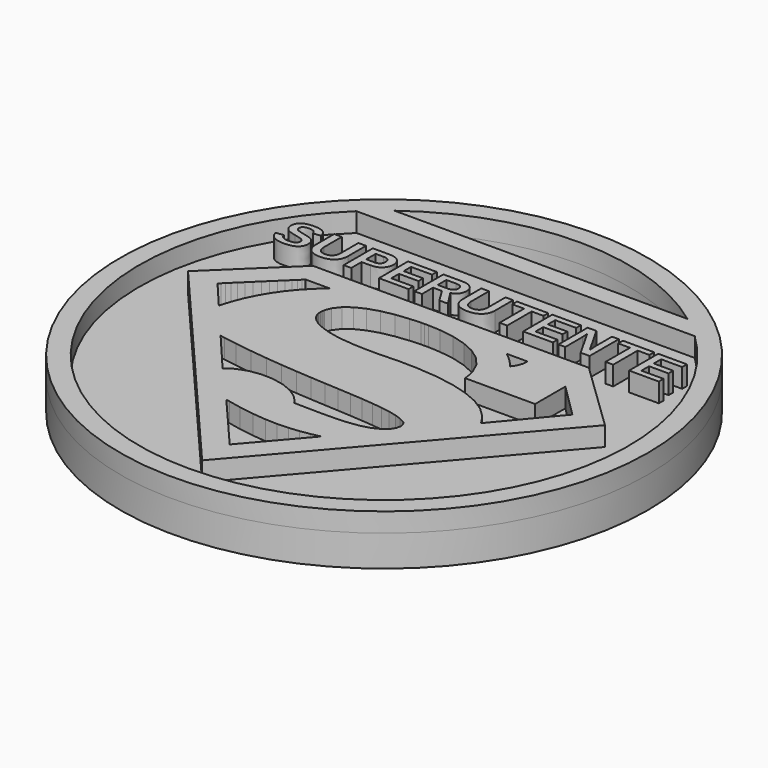
from build123d import *

# Parameters (mm, degrees)
F0_R         = 11
F0_TEXT_SIZE = 2.2071271815
F1_DEPTH     = 1.3
F2_DEPTH     = 0.8


# Not quite as in the source:
# - a feature names something its author has since deleted; it is built from what else it names
# - Text() gives the source's letters only with a copy of the font that has no kerning and outlines rounded to 1/6400 em; it was checked with that copy


with BuildPart() as f1:
    # F0 (on Top) → F1 (new body)
    with BuildSketch(Plane.XY):
        with Locations((0, 3)):
            Circle(F0_R)
        with BuildLine():
            ThreePointArc((7.048873348, 10.3724747896), (0, -7.2), (-7.048873348, 10.3724747896))
            Line((-7.048873348, 10.3724747896), (7.048873348, 10.3724747896))
        make_face(mode=Mode.SUBTRACT)
        with BuildLine():
            Line((6.1033309693, 11.1724752113), (-6.1033309693, 11.1724752113))
            ThreePointArc((-6.1033309693, 11.1724752113), (0, 13.2), (6.1033309693, 11.1724752113))
        make_face(mode=Mode.SUBTRACT)
        with BuildLine():
            Line((7.048873348, 10.3724747896), (-7.048873348, 10.3724747896))
            ThreePointArc((-7.048873348, 10.3724747896), (0, -7.2), (7.048873348, 10.3724747896))
        make_face()
        Polygon((8.687503, 3.64583), (3e-06, -6.47917), (-8.687503, 3.64583), (-5.749997, 6.47917), (5.750003, 6.47917), align=None, mode=Mode.SUBTRACT)
        with BuildLine():
            add(Edge.make_bspline(
                [(-6.856384511, 7.7478548692), (-6.8272435349, 7.6750886449), (-6.8272435349, 7.5802511488)],
                knots=[0, 0, 0, 1, 1, 1], degree=2))
            add(Edge.make_bspline(
                [(-6.8272435349, 7.5802511488), (-6.8272435349, 7.3571243853), (-6.9927780735, 7.2390085947)],
                knots=[0, 0, 0, 1, 1, 1], degree=2))
            add(Edge.make_bspline(
                [(-6.9927780735, 7.2390085947), (-7.1583126121, 7.1208928042), (-7.4783460534, 7.1208928042)],
                knots=[0, 0, 0, 1, 1, 1], degree=2))
            add(Edge.make_bspline(
                [(-7.4783460534, 7.1208928042), (-7.7704455414, 7.1208928042), (-7.9363249436, 7.2245243226)],
                knots=[0, 0, 0, 1, 1, 1], degree=2))
            add(Edge.make_bspline(
                [(-7.9363249436, 7.2245243226), (-8.1022043458, 7.3281558411), (-8.1497955257, 7.5381777869)],
                knots=[0, 0, 0, 1, 1, 1], degree=2))
            Line((-8.1497955257, 7.5381777869), (-7.8425220384, 7.5888727394))
            add(Edge.make_bspline(
                [(-7.8425220384, 7.5888727394), (-7.8111394488, 7.4681704716), (-7.720612748, 7.4136820193)],
                knots=[0, 0, 0, 1, 1, 1], degree=2))
            add(Edge.make_bspline(
                [(-7.720612748, 7.4136820193), (-7.6300860472, 7.3591935671), (-7.4697244629, 7.3591935671)],
                knots=[0, 0, 0, 1, 1, 1], degree=2))
            add(Edge.make_bspline(
                [(-7.4697244629, 7.3591935671), (-7.1365862039, 7.3591935671), (-7.1365862039, 7.5619733769)],
                knots=[0, 0, 0, 1, 1, 1], degree=2))
            add(Edge.make_bspline(
                [(-7.1365862039, 7.5619733769), (-7.1365862039, 7.6264628742), (-7.174866066, 7.6685362361)],
                knots=[0, 0, 0, 1, 1, 1], degree=2))
            add(Edge.make_bspline(
                [(-7.174866066, 7.6685362361), (-7.213145928, 7.710609598), (-7.2826359479, 7.7385435514)],
                knots=[0, 0, 0, 1, 1, 1], degree=2))
            add(Edge.make_bspline(
                [(-7.2826359479, 7.7385435514), (-7.3521259677, 7.7664775048), (-7.5493879596, 7.8064816849)],
                knots=[0, 0, 0, 1, 1, 1], degree=2))
            add(Edge.make_bspline(
                [(-7.5493879596, 7.8064816849), (-7.7197505889, 7.8464858651), (-7.7864816998, 7.8706263186)],
                knots=[0, 0, 0, 1, 1, 1], degree=2))
            add(Edge.make_bspline(
                [(-7.7864816998, 7.8706263186), (-7.8532128107, 7.8947667722), (-7.9071839675, 7.9277012481)],
                knots=[0, 0, 0, 1, 1, 1], degree=2))
            add(Edge.make_bspline(
                [(-7.9071839675, 7.9277012481), (-7.9611551244, 7.960635724), (-7.9987452592, 8.0070198812)],
                knots=[0, 0, 0, 1, 1, 1], degree=2))
            add(Edge.make_bspline(
                [(-7.9987452592, 8.0070198812), (-8.036335394, 8.0534040384), (-8.057372075, 8.115824354)],
                knots=[0, 0, 0, 1, 1, 1], degree=2))
            add(Edge.make_bspline(
                [(-8.057372075, 8.115824354), (-8.0784087559, 8.1782446696), (-8.0784087559, 8.2592876208)],
                knots=[0, 0, 0, 1, 1, 1], degree=2))
            add(Edge.make_bspline(
                [(-8.0784087559, 8.2592876208), (-8.0784087559, 8.4648263395), (-7.9237374214, 8.5743205396)],
                knots=[0, 0, 0, 1, 1, 1], degree=2))
            add(Edge.make_bspline(
                [(-7.9237374214, 8.5743205396), (-7.7690660869, 8.6838147396), (-7.4738628264, 8.6838147396)],
                knots=[0, 0, 0, 1, 1, 1], degree=2))
            add(Edge.make_bspline(
                [(-7.4738628264, 8.6838147396), (-7.1914195198, 8.6838147396), (-7.049853003, 8.5953572205)],
                knots=[0, 0, 0, 1, 1, 1], degree=2))
            add(Edge.make_bspline(
                [(-7.049853003, 8.5953572205), (-6.9082864861, 8.5068997014), (-6.8672477151, 8.3034301644)],
                knots=[0, 0, 0, 1, 1, 1], degree=2))
            Line((-6.8672477151, 8.3034301644), (-7.1755557932, 8.2613568025))
            add(Edge.make_bspline(
                [(-7.1755557932, 8.2613568025), (-7.1990065195, 8.3592980712), (-7.2717727438, 8.4089584328)],
                knots=[0, 0, 0, 1, 1, 1], degree=2))
            add(Edge.make_bspline(
                [(-7.2717727438, 8.4089584328), (-7.3445389681, 8.4586187943), (-7.4804152352, 8.4586187943)],
                knots=[0, 0, 0, 1, 1, 1], degree=2))
            add(Edge.make_bspline(
                [(-7.4804152352, 8.4586187943), (-7.7690660869, 8.4586187943), (-7.7690660869, 8.2775653927)],
                knots=[0, 0, 0, 1, 1, 1], degree=2))
            add(Edge.make_bspline(
                [(-7.7690660869, 8.2775653927), (-7.7690660869, 8.2182488497), (-7.7383732245, 8.1804862831)],
                knots=[0, 0, 0, 1, 1, 1], degree=2))
            add(Edge.make_bspline(
                [(-7.7383732245, 8.1804862831), (-7.7076803621, 8.1427237165), (-7.6473292283, 8.115824354)],
                knots=[0, 0, 0, 1, 1, 1], degree=2))
            add(Edge.make_bspline(
                [(-7.6473292283, 8.115824354), (-7.5869780944, 8.0889249914), (-7.4028209202, 8.0499554021)],
                knots=[0, 0, 0, 1, 1, 1], degree=2))
            add(Edge.make_bspline(
                [(-7.4028209202, 8.0499554021), (-7.1841773838, 8.0037436768), (-7.0898571831, 7.9644292239)],
                knots=[0, 0, 0, 1, 1, 1], degree=2))
            add(Edge.make_bspline(
                [(-7.0898571831, 7.9644292239), (-6.9955369825, 7.9251147709), (-6.9405312348, 7.8728679322)],
                knots=[0, 0, 0, 1, 1, 1], degree=2))
            add(Edge.make_bspline(
                [(-6.9405312348, 7.8728679322), (-6.885525487, 7.8206210934), (-6.856384511, 7.7478548692)],
                knots=[0, 0, 0, 1, 1, 1], degree=2))
        make_face(mode=Mode.SUBTRACT)
        with BuildLine():
            add(Edge.make_bspline(
                [(-5.4602041368, 7.279874934), (-5.6384986295, 7.1208928042), (-5.961980707, 7.1208928042)],
                knots=[0, 0, 0, 1, 1, 1], degree=2))
            add(Edge.make_bspline(
                [(-5.961980707, 7.1208928042), (-6.2754617395, 7.1208928042), (-6.442030869, 7.2740122524)],
                knots=[0, 0, 0, 1, 1, 1], degree=2))
            add(Edge.make_bspline(
                [(-6.442030869, 7.2740122524), (-6.6085999985, 7.4271317006), (-6.6085999985, 7.7116441889)],
                knots=[0, 0, 0, 1, 1, 1], degree=2))
            Line((-6.6085999985, 7.7116441889), (-6.6085999985, 8.6610537405))
            Line((-6.6085999985, 8.6610537405), (-6.2906357389, 8.6610537405))
            Line((-6.2906357389, 8.6610537405), (-6.2906357389, 7.7364743696))
            add(Edge.make_bspline(
                [(-6.2906357389, 7.7364743696), (-6.2906357389, 7.5564555589), (-6.2049371288, 7.4631699491)],
                knots=[0, 0, 0, 1, 1, 1], degree=2))
            add(Edge.make_bspline(
                [(-6.2049371288, 7.4631699491), (-6.1192385187, 7.3698843393), (-5.9533591165, 7.3698843393)],
                knots=[0, 0, 0, 1, 1, 1], degree=2))
            add(Edge.make_bspline(
                [(-5.9533591165, 7.3698843393), (-5.7829964871, 7.3698843393), (-5.6914351955, 7.4674807444)],
                knots=[0, 0, 0, 1, 1, 1], degree=2))
            add(Edge.make_bspline(
                [(-5.6914351955, 7.4674807444), (-5.5998739038, 7.5650771495), (-5.5998739038, 7.7471651419)],
                knots=[0, 0, 0, 1, 1, 1], degree=2))
            Line((-5.5998739038, 7.7471651419), (-5.5998739038, 8.6610537405))
            Line((-5.5998739038, 8.6610537405), (-5.2819096442, 8.6610537405))
            Line((-5.2819096442, 8.6610537405), (-5.2819096442, 7.7278527791))
            add(Edge.make_bspline(
                [(-5.2819096442, 7.7278527791), (-5.2819096442, 7.4388570638), (-5.4602041368, 7.279874934)],
                knots=[0, 0, 0, 1, 1, 1], degree=2))
        make_face(mode=Mode.SUBTRACT)
        with BuildLine():
            add(Edge.make_bspline(
                [(-3.8974546332, 8.5355233821), (-3.7503702984, 8.4099930236), (-3.7503702984, 8.1803138513)],
                knots=[0, 0, 0, 1, 1, 1], degree=2))
            add(Edge.make_bspline(
                [(-3.7503702984, 8.1803138513), (-3.7503702984, 8.0337468119), (-3.8171014093, 7.9185623621)],
                knots=[0, 0, 0, 1, 1, 1], degree=2))
            add(Edge.make_bspline(
                [(-3.8171014093, 7.9185623621), (-3.8838325202, 7.8033779123), (-4.0083282877, 7.7402678695)],
                knots=[0, 0, 0, 1, 1, 1], degree=2))
            add(Edge.make_bspline(
                [(-4.0083282877, 7.7402678695), (-4.1328240553, 7.6771578266), (-4.3042212755, 7.6771578266)],
                knots=[0, 0, 0, 1, 1, 1], degree=2))
            Line((-4.3042212755, 7.6771578266), (-4.6815020781, 7.6771578266))
            Line((-4.6815020781, 7.6771578266), (-4.6815020781, 7.1426192124))
            Line((-4.6815020781, 7.1426192124), (-4.9994663377, 7.1426192124))
            Line((-4.9994663377, 7.1426192124), (-4.9994663377, 8.6610537405))
            Line((-4.9994663377, 8.6610537405), (-4.3173260932, 8.6610537405))
            add(Edge.make_bspline(
                [(-4.3173260932, 8.6610537405), (-4.0445389681, 8.6610537405), (-3.8974546332, 8.5355233821)],
                knots=[0, 0, 0, 1, 1, 1], degree=2))
        make_face(mode=Mode.SUBTRACT)
        Polygon((-2.2888382679, 7.1426192124), (-3.5272435349, 7.1426192124), (-3.5272435349, 8.6610537405), (-2.3329808115, 8.6610537405), (-2.3329808115, 8.4155108416), (-3.2092792753, 8.4155108416), (-3.2092792753, 8.0337468119), (-2.3988497633, 8.0337468119), (-2.3988497633, 7.788203913), (-3.2092792753, 7.788203913), (-3.2092792753, 7.3885069749), (-2.2888382679, 7.3885069749), align=None, mode=Mode.SUBTRACT)
        with BuildLine():
            Line((-0.6538398354, 7.1426192124), (-1.0118082752, 7.1426192124))
            Line((-1.0118082752, 7.1426192124), (-1.364258897, 7.7192311885))
            Line((-1.364258897, 7.7192311885), (-1.7370564725, 7.7192311885))
            Line((-1.7370564725, 7.7192311885), (-1.7370564725, 7.1426192124))
            Line((-1.7370564725, 7.1426192124), (-2.0550207321, 7.1426192124))
            Line((-2.0550207321, 7.1426192124), (-2.0550207321, 8.6610537405))
            Line((-2.0550207321, 8.6610537405), (-1.2963207634, 8.6610537405))
            add(Edge.make_bspline(
                [(-1.2963207634, 8.6610537405), (-1.0245682292, 8.6610537405), (-0.876966599, 8.5441449726)],
                knots=[0, 0, 0, 1, 1, 1], degree=2))
            add(Edge.make_bspline(
                [(-0.876966599, 8.5441449726), (-0.7293649687, 8.4272362047), (-0.7293649687, 8.2085926683)],
                knots=[0, 0, 0, 1, 1, 1], degree=2))
            add(Edge.make_bspline(
                [(-0.7293649687, 8.2085926683), (-0.7293649687, 8.0489208113), (-0.8198916695, 7.9330466342)],
                knots=[0, 0, 0, 1, 1, 1], degree=2))
            add(Edge.make_bspline(
                [(-0.8198916695, 7.9330466342), (-0.9104183703, 7.8171724572), (-1.0645724094, 7.7806169133)],
                knots=[0, 0, 0, 1, 1, 1], degree=2))
            Line((-1.0645724094, 7.7806169133), (-0.6538398354, 7.1426192124))
        make_face(mode=Mode.SUBTRACT)
        with BuildLine():
            add(Edge.make_bspline(
                [(0.6721607916, 7.279874934), (0.4938662989, 7.1208928042), (0.1703842214, 7.1208928042)],
                knots=[0, 0, 0, 1, 1, 1], degree=2))
            add(Edge.make_bspline(
                [(0.1703842214, 7.1208928042), (-0.1430968111, 7.1208928042), (-0.3096659406, 7.2740122524)],
                knots=[0, 0, 0, 1, 1, 1], degree=2))
            add(Edge.make_bspline(
                [(-0.3096659406, 7.2740122524), (-0.4762350701, 7.4271317006), (-0.4762350701, 7.7116441889)],
                knots=[0, 0, 0, 1, 1, 1], degree=2))
            Line((-0.4762350701, 7.7116441889), (-0.4762350701, 8.6610537405))
            Line((-0.4762350701, 8.6610537405), (-0.1582708105, 8.6610537405))
            Line((-0.1582708105, 8.6610537405), (-0.1582708105, 7.7364743696))
            add(Edge.make_bspline(
                [(-0.1582708105, 7.7364743696), (-0.1582708105, 7.5564555589), (-0.0725722004, 7.4631699491)],
                knots=[0, 0, 0, 1, 1, 1], degree=2))
            add(Edge.make_bspline(
                [(-0.0725722004, 7.4631699491), (0.0131264097, 7.3698843393), (0.179005812, 7.3698843393)],
                knots=[0, 0, 0, 1, 1, 1], degree=2))
            add(Edge.make_bspline(
                [(0.179005812, 7.3698843393), (0.3493684413, 7.3698843393), (0.440929733, 7.4674807444)],
                knots=[0, 0, 0, 1, 1, 1], degree=2))
            add(Edge.make_bspline(
                [(0.440929733, 7.4674807444), (0.5324910246, 7.5650771495), (0.5324910246, 7.7471651419)],
                knots=[0, 0, 0, 1, 1, 1], degree=2))
            Line((0.5324910246, 7.7471651419), (0.5324910246, 8.6610537405))
            Line((0.5324910246, 8.6610537405), (0.8504552842, 8.6610537405))
            Line((0.8504552842, 8.6610537405), (0.8504552842, 7.7278527791))
            add(Edge.make_bspline(
                [(0.8504552842, 7.7278527791), (0.8504552842, 7.4388570638), (0.6721607916, 7.279874934)],
                knots=[0, 0, 0, 1, 1, 1], degree=2))
        make_face(mode=Mode.SUBTRACT)
        Polygon((2.309918133, 8.4155108416), (1.8184874715, 8.4155108416), (1.8184874715, 7.1426192124), (1.5005232119, 7.1426192124), (1.5005232119, 8.4155108416), (1.0101271413, 8.4155108416), (1.0101271413, 8.6610537405), (2.309918133, 8.6610537405), align=None, mode=Mode.SUBTRACT)
        Polygon((3.7193757566, 7.1426192124), (2.4809704896, 7.1426192124), (2.4809704896, 8.6610537405), (3.6752332129, 8.6610537405), (3.6752332129, 8.4155108416), (2.7989347492, 8.4155108416), (2.7989347492, 8.0337468119), (3.6093642611, 8.0337468119), (3.6093642611, 7.788203913), (2.7989347492, 7.788203913), (2.7989347492, 7.3885069749), (3.7193757566, 7.3885069749), align=None, mode=Mode.SUBTRACT)
        with BuildLine():
            Line((5.2509151024, 7.1426192124), (4.8777726632, 7.1426192124))
            Line((4.8777726632, 7.1426192124), (4.216324236, 8.312051755))
            add(Edge.make_bspline(
                [(4.216324236, 8.312051755), (4.2356365989, 8.1416891256), (4.2356365989, 8.038230039)],
                knots=[0, 0, 0, 1, 1, 1], degree=2))
            Line((4.2356365989, 8.038230039), (4.2356365989, 7.1426192124))
            Line((4.2356365989, 7.1426192124), (3.9531932924, 7.1426192124))
            Line((3.9531932924, 7.1426192124), (3.9531932924, 8.6610537405))
            Line((3.9531932924, 8.6610537405), (4.3163346864, 8.6610537405))
            Line((4.3163346864, 8.6610537405), (4.9877841587, 7.4819650165))
            add(Edge.make_bspline(
                [(4.9877841587, 7.4819650165), (4.9684717959, 7.6447406462), (4.9684717959, 7.7785477315)],
                knots=[0, 0, 0, 1, 1, 1], degree=2))
            Line((4.9684717959, 7.7785477315), (4.9684717959, 8.6610537405))
            Line((4.9684717959, 8.6610537405), (5.2509151024, 8.6610537405))
            Line((5.2509151024, 8.6610537405), (5.2509151024, 7.1426192124))
        make_face(mode=Mode.SUBTRACT)
        Polygon((6.724172496, 8.4155108416), (6.2327418345, 8.4155108416), (6.2327418345, 7.1426192124), (5.9147775749, 7.1426192124), (5.9147775749, 8.4155108416), (5.4243815043, 8.4155108416), (5.4243815043, 8.6610537405), (6.724172496, 8.6610537405), align=None, mode=Mode.SUBTRACT)
        Polygon((8.1336301196, 7.1426192124), (6.8952248526, 7.1426192124), (6.8952248526, 8.6610537405), (8.089487576, 8.6610537405), (8.089487576, 8.4155108416), (7.2131891122, 8.4155108416), (7.2131891122, 8.0337468119), (8.0236186242, 8.0337468119), (8.0236186242, 7.788203913), (7.2131891122, 7.788203913), (7.2131891122, 7.3885069749), (8.1336301196, 7.3885069749), align=None, mode=Mode.SUBTRACT)
        Polygon((-8.687503, 3.64583), (3e-06, -6.47917), (8.687503, 3.64583), (5.750003, 6.47917), (-5.749997, 6.47917), align=None)
        Polygon((3e-06, -5.04177), (-2.065417, -2.63737), (-1.895277, -2.67753), (-1.380757, -2.78189), (-0.763557, -2.87825), (-0.205717, -2.93165), (0.300783, -2.94737), (0.764223, -2.93079), (1.192723, -2.88705), (1.594383, -2.82161), (1.882163, -2.76205), (1.977523, -2.73969), align=None, mode=Mode.SUBTRACT)
        Polygon((-3.531257, -1.00001), (-5.021917, 0.76183), (-4.839077, 0.72853), (-4.288317, 0.63889), (-3.567817, 0.53809), (-2.863717, 0.45617), (-2.178817, 0.39019), (-1.516397, 0.33713), (-0.879557, 0.29383), (-0.271177, 0.25727), (0.305443, 0.22439), (0.847443, 0.19217), (1.351543, 0.15745), (1.814883, 0.11719), (2.234163, 0.06847), (2.606443, 0.00791), (2.928603, -0.06729), (3.197683, -0.16029), (3.360883, -0.24023), (3.410463, -0.27409), (3.443803, -0.30015), (3.520603, -0.40843), (3.549363, -0.56283), (3.510083, -0.72775), (3.444003, -0.85525), (3.416663, -0.89401), (3.365443, -0.95595), (3.172523, -1.10929), (2.855143, -1.26401), (2.471663, -1.36761), (2.028963, -1.42947), (1.534163, -1.45897), (0.994243, -1.46561), (0.416223, -1.45879), (-0.040477, -1.45031), (-0.192697, -1.44791), (-0.248057, -1.35275), (-0.474277, -1.10241), (-0.851457, -0.83811), (-1.295997, -0.65551), (-1.779317, -0.55567), (-2.272897, -0.53929), (-2.748477, -0.60731), (-3.177417, -0.76065), (-3.453677, -0.92839), align=None, mode=Mode.SUBTRACT)
        Polygon((-6.387357, 2.37575), (-7.395837, 3.56771), (-7.376089, 3.58953), (-7.313037, 3.65267), (-7.212797, 3.75141), (-7.081497, 3.87967), (-6.925357, 4.03169), (-6.750657, 4.20161), (-6.563257, 4.38335), (-6.369477, 4.57097), (-6.175557, 4.75877), (-5.987417, 4.94063), (-5.811417, 5.11089), (-5.653637, 5.26333), (-5.520197, 5.39225), (-5.417217, 5.49153), (-5.351037, 5.55555), (-5.327477, 5.57813), (-4.317697, 5.57813), (-4.413837, 5.50131), (-4.689457, 5.25489), (-5.031137, 4.90471), (-5.341817, 4.53005), (-5.619997, 4.13347), (-5.864917, 3.71721), (-6.075197, 3.28397), (-6.249777, 2.83605), (-6.357757, 2.49207), align=None, mode=Mode.SUBTRACT)
        Polygon((7.395823, 3.56771), (5.442803, 1.23155), (5.386383, 1.34397), (5.165243, 1.65483), (4.786463, 2.02117), (4.306423, 2.32963), (3.725363, 2.57963), (3.043603, 2.77039), (2.261283, 2.90113), (1.378583, 2.97103), (0.641283, 2.98459), (0.395823, 2.97917), (0.242083, 2.97147), (-0.219717, 2.95833), (-0.770717, 2.96007), (-1.260537, 2.98219), (-1.692177, 3.02277), (-2.068897, 3.07975), (-2.394077, 3.15105), (-2.670777, 3.23447), (-2.902217, 3.32821), (-3.091577, 3.43011), (-3.242197, 3.53809), (-3.357197, 3.64995), (-3.439897, 3.76389), (-3.493277, 3.87771), (-3.520717, 3.98935), (-3.525397, 4.09677), (-3.516497, 4.17327), (-3.510417, 4.19791), (-3.498917, 4.28027), (-3.405497, 4.51919), (-3.194777, 4.79439), (-2.889857, 5.02505), (-2.502177, 5.21213), (-2.043197, 5.35709), (-1.524197, 5.46117), (-0.956817, 5.52549), (-0.503577, 5.54959), (-0.352417, 5.55121), (-0.187717, 5.55305), (0.307183, 5.52681), (0.928723, 5.43675), (1.497943, 5.27885), (2.000323, 5.05089), (2.421663, 4.75045), (2.747603, 4.37533), (2.963643, 3.92327), (3.049923, 3.52549), (3.055783, 3.39191), (5.979903, 3.39191), (5.979903, 4.96819), align=None, mode=Mode.SUBTRACT)
        Polygon((3.065963, 5.56119), (3.036463, 5.57813), (3.911463, 5.57813), (3.914723, 5.52397), (3.896923, 5.35959), (3.838963, 5.18295), (3.759323, 5.04719), (3.700943, 4.97385), (3.679583, 4.95139), (3.640723, 5.00639), (3.509783, 5.16125), (3.325943, 5.34733), (3.158083, 5.49219), align=None, mode=Mode.SUBTRACT)
        Polygon((5.386383, 1.34397), (5.442803, 1.23155), (7.395823, 3.56771), (5.979903, 4.96819), (5.979903, 3.39191), (3.055783, 3.39191), (3.049923, 3.52549), (2.963643, 3.92327), (2.747603, 4.37533), (2.421663, 4.75045), (2.000323, 5.05089), (1.497943, 5.27885), (0.928723, 5.43675), (0.307183, 5.52681), (-0.187717, 5.55305), (-0.352417, 5.55121), (-0.503577, 5.54959), (-0.956817, 5.52549), (-1.524197, 5.46117), (-2.043197, 5.35709), (-2.502177, 5.21213), (-2.889857, 5.02505), (-3.194777, 4.79439), (-3.405497, 4.51919), (-3.498917, 4.28027), (-3.510417, 4.19791), (-3.516497, 4.17327), (-3.525397, 4.09677), (-3.520717, 3.98935), (-3.493277, 3.87771), (-3.439897, 3.76389), (-3.357197, 3.64995), (-3.242197, 3.53809), (-3.091577, 3.43011), (-2.902217, 3.32821), (-2.670777, 3.23447), (-2.394077, 3.15105), (-2.068897, 3.07975), (-1.692177, 3.02277), (-1.260537, 2.98219), (-0.770717, 2.96007), (-0.219717, 2.95833), (0.242083, 2.97147), (0.395823, 2.97917), (0.641283, 2.98459), (1.378583, 2.97103), (2.261283, 2.90113), (3.043603, 2.77039), (3.725363, 2.57963), (4.306423, 2.32963), (4.786463, 2.02117), (5.165243, 1.65483), align=None)
        Polygon((-4.839077, 0.72853), (-5.021917, 0.76183), (-3.531257, -1.00001), (-3.453677, -0.92839), (-3.177417, -0.76065), (-2.748477, -0.60731), (-2.272897, -0.53929), (-1.779317, -0.55567), (-1.295997, -0.65551), (-0.851457, -0.83811), (-0.474277, -1.10241), (-0.248057, -1.35275), (-0.192697, -1.44791), (-0.040477, -1.45031), (0.416223, -1.45879), (0.994243, -1.46561), (1.534163, -1.45897), (2.028963, -1.42947), (2.471663, -1.36761), (2.855143, -1.26401), (3.172523, -1.10929), (3.365443, -0.95595), (3.416663, -0.89401), (3.444003, -0.85525), (3.510083, -0.72775), (3.549363, -0.56283), (3.520603, -0.40843), (3.443803, -0.30015), (3.410463, -0.27409), (3.360883, -0.24023), (3.197683, -0.16029), (2.928603, -0.06729), (2.606443, 0.00791), (2.234163, 0.06847), (1.814883, 0.11719), (1.351543, 0.15745), (0.847443, 0.19217), (0.305443, 0.22439), (-0.271177, 0.25727), (-0.879557, 0.29383), (-1.516397, 0.33713), (-2.178817, 0.39019), (-2.863717, 0.45617), (-3.567817, 0.53809), (-4.288317, 0.63889), align=None)
        Polygon((-1.895277, -2.67753), (-2.065417, -2.63737), (3e-06, -5.04177), (1.977523, -2.73969), (1.882163, -2.76205), (1.594383, -2.82161), (1.192723, -2.88705), (0.764223, -2.93079), (0.300783, -2.94737), (-0.205717, -2.93165), (-0.763557, -2.87825), (-1.380757, -2.78189), align=None)
        Polygon((-7.376089, 3.58953), (-7.395837, 3.56771), (-6.387357, 2.37575), (-6.357757, 2.49207), (-6.249777, 2.83605), (-6.075197, 3.28397), (-5.864917, 3.71721), (-5.619997, 4.13347), (-5.341817, 4.53005), (-5.031137, 4.90471), (-4.689457, 5.25489), (-4.413837, 5.50131), (-4.317697, 5.57813), (-5.327477, 5.57813), (-5.351037, 5.55555), (-5.417217, 5.49153), (-5.520197, 5.39225), (-5.653637, 5.26333), (-5.811417, 5.11089), (-5.987417, 4.94063), (-6.175557, 4.75877), (-6.369477, 4.57097), (-6.563257, 4.38335), (-6.750657, 4.20161), (-6.925357, 4.03169), (-7.081497, 3.87967), (-7.212797, 3.75141), (-7.313037, 3.65267), align=None)
        with Locations((-8.2132504322, 7.1426192124)):
            Text('SUPERUTENTE', F0_TEXT_SIZE, font='Arimo', font_style=FontStyle.BOLD, text_align=(TextAlign.LEFT, TextAlign.BOTTOM))
        with BuildLine():
            add(Edge.make_bspline(
                [(-1.1183711344, 8.0265046758), (-1.04939841, 8.0868558097), (-1.04939841, 8.1954878507)],
                knots=[0, 0, 0, 1, 1, 1], degree=2))
            add(Edge.make_bspline(
                [(-1.04939841, 8.1954878507), (-1.04939841, 8.4144762507), (-1.3297725348, 8.4144762507)],
                knots=[0, 0, 0, 1, 1, 1], degree=2))
            Line((-1.3297725348, 8.4144762507), (-1.7370564725, 8.4144762507))
            Line((-1.7370564725, 8.4144762507), (-1.7370564725, 7.966153542))
            Line((-1.7370564725, 7.966153542), (-1.3211509442, 7.966153542))
            add(Edge.make_bspline(
                [(-1.3211509442, 7.966153542), (-1.1873438589, 7.966153542), (-1.1183711344, 8.0265046758)],
                knots=[0, 0, 0, 1, 1, 1], degree=2))
        make_face()
        Polygon((3.911463, 5.57813), (3.036463, 5.57813), (3.065963, 5.56119), (3.158083, 5.49219), (3.325943, 5.34733), (3.509783, 5.16125), (3.640723, 5.00639), (3.679583, 4.95139), (3.700943, 4.97385), (3.759323, 5.04719), (3.838963, 5.18295), (3.896923, 5.35959), (3.914723, 5.52397), align=None)
        with BuildLine():
            add(Edge.make_bspline(
                [(-4.1416180777, 7.9870177911), (-4.0704037397, 8.0523694475), (-4.0704037397, 8.175140897)],
                knots=[0, 0, 0, 1, 1, 1], degree=2))
            add(Edge.make_bspline(
                [(-4.0704037397, 8.175140897), (-4.0704037397, 8.4144762507), (-4.3528470462, 8.4144762507)],
                knots=[0, 0, 0, 1, 1, 1], degree=2))
            Line((-4.3528470462, 8.4144762507), (-4.6815020781, 8.4144762507))
            Line((-4.6815020781, 8.4144762507), (-4.6815020781, 7.9216661347))
            Line((-4.6815020781, 7.9216661347), (-4.3442254557, 7.9216661347))
            add(Edge.make_bspline(
                [(-4.3442254557, 7.9216661347), (-4.2128324157, 7.9216661347), (-4.1416180777, 7.9870177911)],
                knots=[0, 0, 0, 1, 1, 1], degree=2))
        make_face()
    extrude(amount=-F1_DEPTH)

    # F0 (on Top) → F2 (join)
    with BuildSketch(Plane.XY):
        with Locations((0, 3)):
            Circle(F0_R)
        with BuildLine():
            ThreePointArc((7.048873348, 10.3724747896), (0, -7.2), (-7.048873348, 10.3724747896))
            Line((-7.048873348, 10.3724747896), (7.048873348, 10.3724747896))
        make_face(mode=Mode.SUBTRACT)
        with BuildLine():
            Line((6.1033309693, 11.1724752113), (-6.1033309693, 11.1724752113))
            ThreePointArc((-6.1033309693, 11.1724752113), (0, 13.2), (6.1033309693, 11.1724752113))
        make_face(mode=Mode.SUBTRACT)
        Polygon((-8.687503, 3.64583), (3e-06, -6.47917), (8.687503, 3.64583), (5.750003, 6.47917), (-5.749997, 6.47917), align=None)
        Polygon((3e-06, -5.04177), (-2.065417, -2.63737), (-1.895277, -2.67753), (-1.380757, -2.78189), (-0.763557, -2.87825), (-0.205717, -2.93165), (0.300783, -2.94737), (0.764223, -2.93079), (1.192723, -2.88705), (1.594383, -2.82161), (1.882163, -2.76205), (1.977523, -2.73969), align=None, mode=Mode.SUBTRACT)
        Polygon((-3.531257, -1.00001), (-5.021917, 0.76183), (-4.839077, 0.72853), (-4.288317, 0.63889), (-3.567817, 0.53809), (-2.863717, 0.45617), (-2.178817, 0.39019), (-1.516397, 0.33713), (-0.879557, 0.29383), (-0.271177, 0.25727), (0.305443, 0.22439), (0.847443, 0.19217), (1.351543, 0.15745), (1.814883, 0.11719), (2.234163, 0.06847), (2.606443, 0.00791), (2.928603, -0.06729), (3.197683, -0.16029), (3.360883, -0.24023), (3.410463, -0.27409), (3.443803, -0.30015), (3.520603, -0.40843), (3.549363, -0.56283), (3.510083, -0.72775), (3.444003, -0.85525), (3.416663, -0.89401), (3.365443, -0.95595), (3.172523, -1.10929), (2.855143, -1.26401), (2.471663, -1.36761), (2.028963, -1.42947), (1.534163, -1.45897), (0.994243, -1.46561), (0.416223, -1.45879), (-0.040477, -1.45031), (-0.192697, -1.44791), (-0.248057, -1.35275), (-0.474277, -1.10241), (-0.851457, -0.83811), (-1.295997, -0.65551), (-1.779317, -0.55567), (-2.272897, -0.53929), (-2.748477, -0.60731), (-3.177417, -0.76065), (-3.453677, -0.92839), align=None, mode=Mode.SUBTRACT)
        Polygon((-6.387357, 2.37575), (-7.395837, 3.56771), (-7.376089, 3.58953), (-7.313037, 3.65267), (-7.212797, 3.75141), (-7.081497, 3.87967), (-6.925357, 4.03169), (-6.750657, 4.20161), (-6.563257, 4.38335), (-6.369477, 4.57097), (-6.175557, 4.75877), (-5.987417, 4.94063), (-5.811417, 5.11089), (-5.653637, 5.26333), (-5.520197, 5.39225), (-5.417217, 5.49153), (-5.351037, 5.55555), (-5.327477, 5.57813), (-4.317697, 5.57813), (-4.413837, 5.50131), (-4.689457, 5.25489), (-5.031137, 4.90471), (-5.341817, 4.53005), (-5.619997, 4.13347), (-5.864917, 3.71721), (-6.075197, 3.28397), (-6.249777, 2.83605), (-6.357757, 2.49207), align=None, mode=Mode.SUBTRACT)
        Polygon((7.395823, 3.56771), (5.442803, 1.23155), (5.386383, 1.34397), (5.165243, 1.65483), (4.786463, 2.02117), (4.306423, 2.32963), (3.725363, 2.57963), (3.043603, 2.77039), (2.261283, 2.90113), (1.378583, 2.97103), (0.641283, 2.98459), (0.395823, 2.97917), (0.242083, 2.97147), (-0.219717, 2.95833), (-0.770717, 2.96007), (-1.260537, 2.98219), (-1.692177, 3.02277), (-2.068897, 3.07975), (-2.394077, 3.15105), (-2.670777, 3.23447), (-2.902217, 3.32821), (-3.091577, 3.43011), (-3.242197, 3.53809), (-3.357197, 3.64995), (-3.439897, 3.76389), (-3.493277, 3.87771), (-3.520717, 3.98935), (-3.525397, 4.09677), (-3.516497, 4.17327), (-3.510417, 4.19791), (-3.498917, 4.28027), (-3.405497, 4.51919), (-3.194777, 4.79439), (-2.889857, 5.02505), (-2.502177, 5.21213), (-2.043197, 5.35709), (-1.524197, 5.46117), (-0.956817, 5.52549), (-0.503577, 5.54959), (-0.352417, 5.55121), (-0.187717, 5.55305), (0.307183, 5.52681), (0.928723, 5.43675), (1.497943, 5.27885), (2.000323, 5.05089), (2.421663, 4.75045), (2.747603, 4.37533), (2.963643, 3.92327), (3.049923, 3.52549), (3.055783, 3.39191), (5.979903, 3.39191), (5.979903, 4.96819), align=None, mode=Mode.SUBTRACT)
        Polygon((3.065963, 5.56119), (3.036463, 5.57813), (3.911463, 5.57813), (3.914723, 5.52397), (3.896923, 5.35959), (3.838963, 5.18295), (3.759323, 5.04719), (3.700943, 4.97385), (3.679583, 4.95139), (3.640723, 5.00639), (3.509783, 5.16125), (3.325943, 5.34733), (3.158083, 5.49219), align=None, mode=Mode.SUBTRACT)
        with Locations((-8.2132504322, 7.1426192124)):
            Text('SUPERUTENTE', F0_TEXT_SIZE, font='Arimo', font_style=FontStyle.BOLD, text_align=(TextAlign.LEFT, TextAlign.BOTTOM))
    extrude(amount=F2_DEPTH)


solid = f1.part
